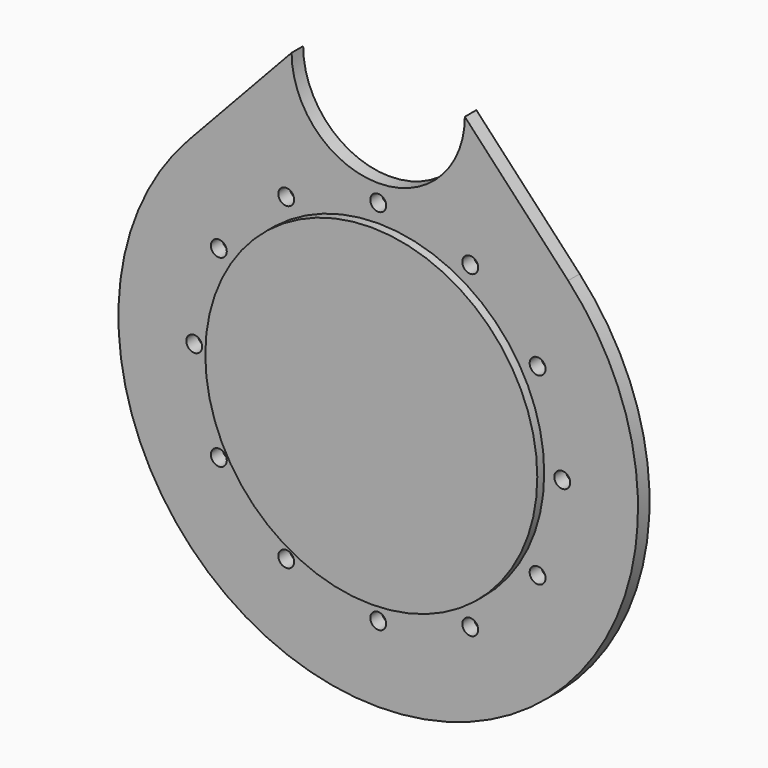
from build123d import *

# Parameters (mm, degrees)
F1_DEPTH = 10
F3_DEPTH = 10
F4_R     = 115
F5_DEPTH = 6
F6_R     = 5.5
F7_DEPTH = 10


with BuildPart() as f1:
    # F0 (on Front) → F1 (new body)
    with BuildSketch(Plane.XZ):
        with BuildLine():
            Line((-60, 199.5), (-131.5733290036, 122.8350890215))
            ThreePointArc((-131.5733290036, 122.8350890215), (0, -180), (131.5733290036, 122.8350890215))
            Line((131.5733290036, 122.8350890215), (60, 199.5))
            Line((60, 199.5), (0, 199.5))
            Line((0, 199.5), (-60, 199.5))
        make_face()
    extrude(amount=-F1_DEPTH)

    # F2 (on face) → F3 (cut, through all)
    with BuildSketch(Plane.XZ):
        with BuildLine():
            Line((-60, 199.5), (60, 199.5))
            ThreePointArc((60, 199.5), (0, 259.5), (-60, 199.5))
        make_face()
        with BuildLine():
            ThreePointArc((-60, 199.5), (0, 139.5), (60, 199.5))
            Line((60, 199.5), (-60, 199.5))
        make_face()
    extrude(amount=-F3_DEPTH, mode=Mode.SUBTRACT)

    # F4 (on face) → F5 (join)
    with BuildSketch(Plane.XZ):
        Circle(F4_R)
    extrude(amount=F5_DEPTH)

    # F6 (on face) → F7 (cut, through all)
    with BuildSketch(Plane.XZ):
        with Locations((-63.75, 110.4182389825)):
            Circle(F6_R)
        with Locations((0, 127.5)):
            Circle(F6_R)
        with Locations((63.75, 110.4182389825)):
            Circle(F6_R)
        with Locations((110.4182389825, 63.75)):
            Circle(F6_R)
        with Locations((127.5, 0)):
            Circle(F6_R)
        with Locations((110.4182389825, -63.75)):
            Circle(F6_R)
        with Locations((63.75, -110.4182389825)):
            Circle(F6_R)
        with Locations((0, -127.5)):
            Circle(F6_R)
        with Locations((-63.75, -110.4182389825)):
            Circle(F6_R)
        with Locations((-110.4182389825, -63.75)):
            Circle(F6_R)
        with Locations((-127.5, 0)):
            Circle(F6_R)
        with Locations((-110.4182389825, 63.75)):
            Circle(F6_R)
    extrude(amount=-F7_DEPTH, mode=Mode.SUBTRACT)


solid = f1.part
